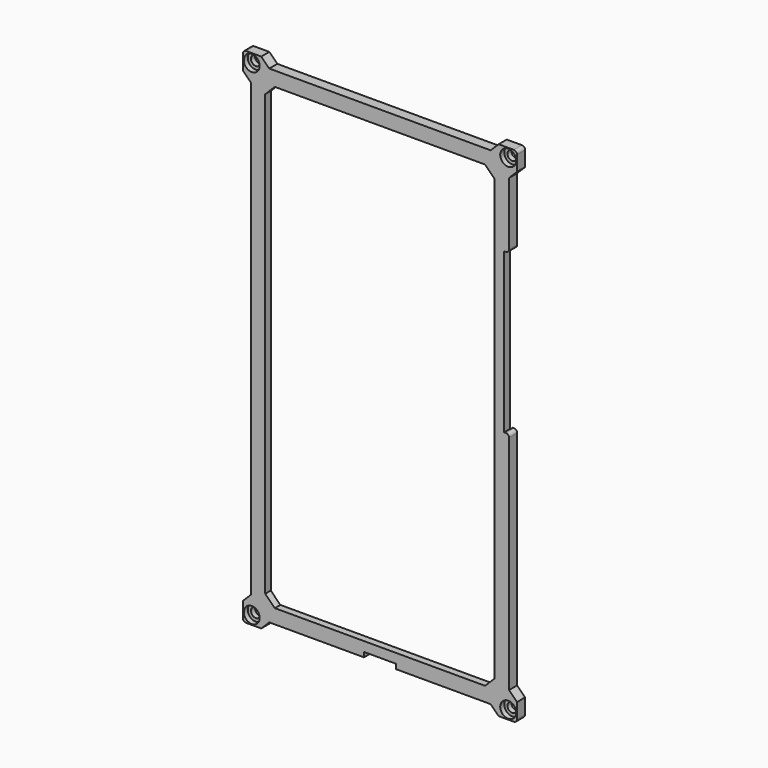
from build123d import *

# Parameters (mm, degrees)
F1_R     = 1.5
F1_W     = 72
F1_H     = 144
F2_DEPTH = 3.175
F3_SIZE  = 3
F4_SIZE  = 2.49999
F5_R     = 1
F6_R     = 2.5
F7_DEPTH = 1.5875
F8_W     = 78.25
F8_H     = 150.25
F9_DEPTH = 1


# Not quite as in the source:
# - a fillet or chamfer is up to 0.001 mm smaller than in the source, because OpenCascade refuses the exact size


with BuildPart() as f2:
    # F1 (on Front) → F2 (new body)
    with BuildSketch(Plane.XZ):
        Polygon((43, 73.2426406871), (43, 79), (37.2426406871, 79), (37.2426406871, 76.5), (-37.2426406871, 76.5), (-37.2426406871, 79), (-43, 79), (-43, 73.2426406871), (-40.5, 73.2426406871), (-40.5, -73.2426406871), (-43, -73.2426406871), (-43, -79), (-37.2426406871, -79), (-37.2426406871, -76.5), (-5, -76.5), (-5, -75), (5, -75), (5, -76.5), (37.2426406871, -76.5), (37.2426406871, -79), (43, -79), (43, -73.2426406871), (40.5, -73.2426406871), (40.5, 0), (39, 0), (39, 50), (40.5, 50), (40.5, 73.2426406871), align=None)
        with Locations((-40.2426406871, -76.2426406871)):
            Circle(F1_R, mode=Mode.SUBTRACT)
        with Locations((40.2426406871, -76.2426406871)):
            Circle(F1_R, mode=Mode.SUBTRACT)
        with Locations((-40.2426406871, 76.2426406871)):
            Circle(F1_R, mode=Mode.SUBTRACT)
        Rectangle(F1_W, F1_H, mode=Mode.SUBTRACT)
        with Locations((40.2426406871, 76.2426406871)):
            Circle(F1_R, mode=Mode.SUBTRACT)
    extrude(amount=F2_DEPTH)

    # F3
    f3_edges = [f2.edges().sort_by_distance(p)[0] for p in [
        (-36, -1.5875, 72),
        (36, -1.5875, 72),
        (36, -1.5875, -72),
        (-36, -1.5875, -72),
    ]]
    chamfer(f3_edges, length=F3_SIZE)

    # F4 (size 2.5 in the source; OpenCascade refuses exactly that, so slightly less here)
    f4_edges = [f2.edges().sort_by_distance(p)[0] for p in [
        (-37.242641, -1.5875, 76.5),
        (-40.5, -1.5875, 73.242641),
        (40.5, -1.5875, 73.242641),
        (37.242641, -1.5875, 76.5),
        (37.242641, -1.5875, -76.5),
        (40.5, -1.5875, -73.242641),
        (-40.5, -1.5875, -73.242641),
        (-37.242641, -1.5875, -76.5),
    ]]
    chamfer(f4_edges, length=F4_SIZE)

    # F5
    f5_edges = [f2.edges().sort_by_distance(p)[0] for p in [
        (-43, -1.5875, 79),
        (43, -1.5875, 79),
        (43, -1.5875, -79),
        (-43, -1.5875, -79),
        (40.5, -1.5875, 0),
        (40.5, -1.5875, 50),
    ]]
    fillet(f5_edges, radius=F5_R)

    # F6 (on face) → F7 (cut)
    with BuildSketch(Plane.XZ.offset(3.175)):
        with Locations((-40.2426406871, 76.2426406871)):
            Circle(F6_R)
        with Locations((40.2426406871, 76.2426406871)):
            Circle(F6_R)
        with Locations((40.2426406871, -76.2426406871)):
            Circle(F6_R)
        with Locations((-40.2426406871, -76.2426406871)):
            Circle(F6_R)
    extrude(amount=-F7_DEPTH, mode=Mode.SUBTRACT)

    # F8 (on face) → F9 (cut)
    with BuildSketch(Plane.XZ):
        Rectangle(F8_W, F8_H)
    extrude(amount=F9_DEPTH, mode=Mode.SUBTRACT)


solid = f2.part
